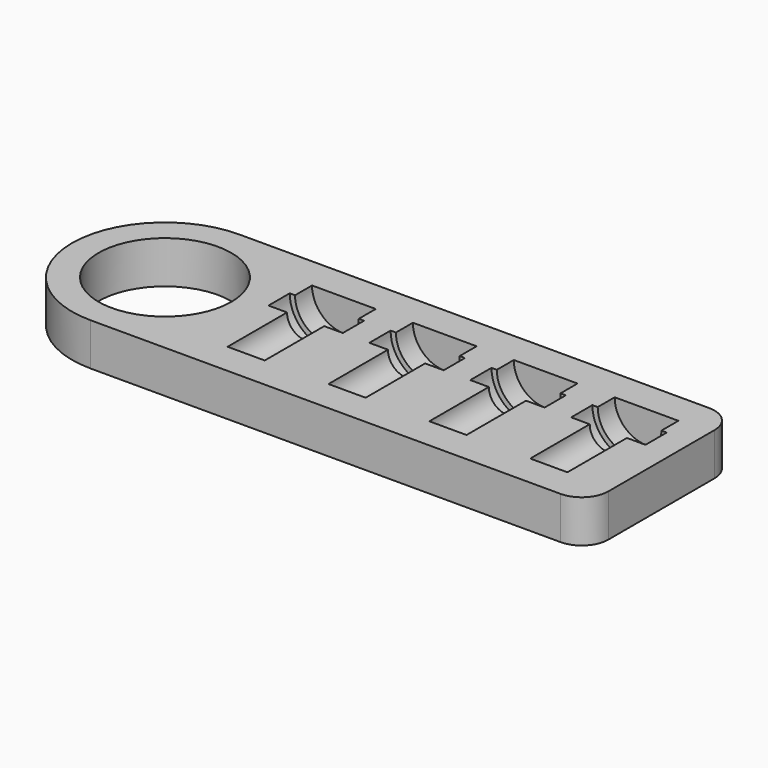
from build123d import *

# Parameters (mm, degrees)
F0_R         = 12.5
F1_DEPTH     = 8
F7_TEXT_SIZE = 5.5555555556
F8_DEPTH     = 1


# Not quite as in the source:
# - Text() gives the source's letters only with a copy of the font that has no kerning and outlines rounded to 1/6400 em; it was checked with that copy


with BuildPart() as f1:
    # F0 (on Top) → F1 (new body)
    with BuildSketch(Plane.XY):
        with BuildLine():
            ThreePointArc((0, 17.5), (5.1256313292, 5.1256313292), (17.5, 0))
            Line((17.5, 0), (106, 0))
            ThreePointArc((106, 0), (109.5355339059, 1.4644660941), (111, 5))
            Line((111, 5), (111, 30))
            ThreePointArc((111, 30), (109.5355339059, 33.5355339059), (106, 35))
            Line((106, 35), (17.5, 35))
            ThreePointArc((17.5, 35), (5.1256313292, 29.8743686708), (0, 17.5))
        make_face()
        with Locations((17.5, 17.5)):
            Circle(F0_R, mode=Mode.SUBTRACT)
    extrude(amount=F1_DEPTH)

    # F2 (on face) → F3 (revolve, cut)
    with BuildSketch(Plane.XY.offset(8)):
        Polygon((42, 20), (42, 6), (45.5, 6), (45.5, 20), (49, 20), (49, 25), (48, 25), (48, 29), (42, 29), (42, 25), align=None)
    revolve(axis=Axis((42, 22.5, 8), (0, 1, 0)), mode=Mode.SUBTRACT)

    # F2 (on face) → F4 (revolve, cut)
    with BuildSketch(Plane.XY.offset(8)):
        Polygon((61, 20), (61, 6), (64.5, 6), (64.5, 20), (68, 20), (68, 25), (67, 25), (67, 29), (61, 29), (61, 25), align=None)
    revolve(axis=Axis((61, 22.5, 8), (0, 1, 0)), mode=Mode.SUBTRACT)

    # F2 (on face) → F5 (revolve, cut)
    with BuildSketch(Plane.XY.offset(8)):
        Polygon((80, 20), (80, 6), (83.5, 6), (83.5, 20), (87, 20), (87, 25), (86, 25), (86, 29), (80, 29), (80, 25), align=None)
    revolve(axis=Axis((80, 13, 8), (0, 1, 0)), mode=Mode.SUBTRACT)

    # F2 (on face) → F6 (revolve, cut)
    with BuildSketch(Plane.XY.offset(8)):
        Polygon((99, 20), (99, 6), (102.5, 6), (102.5, 20), (106, 20), (106, 25), (105, 25), (105, 29), (99, 29), (99, 25), align=None)
    revolve(axis=Axis((99, 13, 8), (0, 1, 0)), mode=Mode.SUBTRACT)

    # F7 (on face) → F8 (cut)
    with BuildSketch(Plane(origin=(0, 0, 0), x_dir=(1, 0, 0), z_dir=(0, 0, -1))):
        with Locations((30, -9)):
            Text('1029', F7_TEXT_SIZE, font='Open Sans', text_align=(TextAlign.LEFT, TextAlign.BOTTOM))
    extrude(amount=-F8_DEPTH, mode=Mode.SUBTRACT)


solid = f1.part
